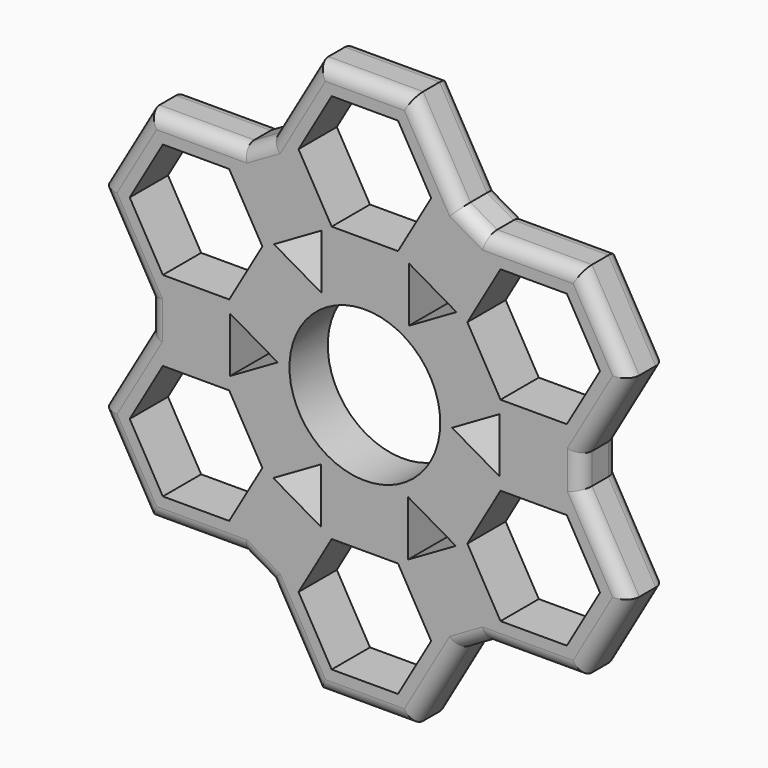
from build123d import *

# Parameters (mm, degrees)
F0_R     = 14.5
F0_R_2   = 11.025
F1_DEPTH = 7
F2_R     = 2
F4_DEPTH = 7


# Not quite as in the source:
# - a feature names something its author has since deleted; it is built from what else it names


with BuildPart() as f1:
    # F0 (on Front) → F1 (new body)
    with BuildSketch(Plane.XZ):
        Polygon((13.8564064606, 28.5096937621), (6.9282032303, 16.5096937621), (-6.9282032303, 16.5096937621), (-13.8564064606, 28.5096937621), (-17.7619158218, 26.254846881), (-10.8337125915, 14.254846881), (-17.7619158218, 2.254846881), (-31.6183222823, 2.254846881), (-31.6183222823, -2.254846881), (-17.7619158218, -2.254846881), (-10.8337125915, -14.254846881), (-17.7619158218, -26.254846881), (-13.8564064606, -28.5096937621), (-6.9282032303, -16.5096937621), (6.9282032303, -16.5096937621), (13.8564064606, -28.5096937621), (17.7619158218, -26.254846881), (10.8337125915, -14.254846881), (17.7619158218, -2.254846881), (31.6183222823, -2.254846881), (31.6183222823, 2.254846881), (17.7619158218, 2.254846881), (10.8337125915, 14.254846881), (17.7619158218, 26.254846881), align=None)
        Circle(F0_R, mode=Mode.SUBTRACT)
        Polygon((-6.9282032303, 16.5096937621), (6.9282032303, 16.5096937621), (13.8564064606, 28.5096937621), (6.9282032303, 40.5096937621), (-6.9282032303, 40.5096937621), (-13.8564064606, 28.5096937621), align=None)
        Polygon((9.6994845224, 28.5096937621), (4.8497422612, 20.1096937621), (-4.8497422612, 20.1096937621), (-9.6994845224, 28.5096937621), (-4.8497422612, 36.9096937621), (4.8497422612, 36.9096937621), align=None, mode=Mode.SUBTRACT)
        Polygon((31.6183222823, 26.254846881), (17.7619158218, 26.254846881), (10.8337125915, 14.254846881), (17.7619158218, 2.254846881), (31.6183222823, 2.254846881), (38.5465255126, 14.254846881), align=None)
        Polygon((29.5398613133, 22.654846881), (34.3896035744, 14.254846881), (29.5398613133, 5.854846881), (19.8403767909, 5.854846881), (14.9906345297, 14.254846881), (19.8403767909, 22.654846881), align=None, mode=Mode.SUBTRACT)
        Polygon((-10.8337125915, 14.254846881), (-17.7619158218, 26.254846881), (-31.6183222823, 26.254846881), (-38.5465255126, 14.254846881), (-31.6183222823, 2.254846881), (-17.7619158218, 2.254846881), align=None)
        Polygon((-34.3896035744, 14.254846881), (-29.5398613133, 22.654846881), (-19.8403767909, 22.654846881), (-14.9906345297, 14.254846881), (-19.8403767909, 5.854846881), (-29.5398613133, 5.854846881), align=None, mode=Mode.SUBTRACT)
        Polygon((38.5465255126, -14.254846881), (31.6183222823, -2.254846881), (17.7619158218, -2.254846881), (10.8337125915, -14.254846881), (17.7619158218, -26.254846881), (31.6183222823, -26.254846881), align=None)
        Polygon((34.3896035744, -14.254846881), (29.5398613133, -22.654846881), (19.8403767909, -22.654846881), (14.9906345297, -14.254846881), (19.8403767909, -5.854846881), (29.5398613133, -5.854846881), align=None, mode=Mode.SUBTRACT)
        Polygon((-17.7619158218, -2.254846881), (-31.6183222823, -2.254846881), (-38.5465255126, -14.254846881), (-31.6183222823, -26.254846881), (-17.7619158218, -26.254846881), (-10.8337125915, -14.254846881), align=None)
        Polygon((-29.5398613133, -22.654846881), (-34.3896035744, -14.254846881), (-29.5398613133, -5.854846881), (-19.8403767909, -5.854846881), (-14.9906345297, -14.254846881), (-19.8403767909, -22.654846881), align=None, mode=Mode.SUBTRACT)
        Polygon((6.9282032303, -40.5096937621), (13.8564064606, -28.5096937621), (6.9282032303, -16.5096937621), (-6.9282032303, -16.5096937621), (-13.8564064606, -28.5096937621), (-6.9282032303, -40.5096937621), align=None)
        Polygon((4.8497422612, -36.9096937621), (-4.8497422612, -36.9096937621), (-9.6994845224, -28.5096937621), (-4.8497422612, -20.1096937621), (4.8497422612, -20.1096937621), (9.6994845224, -28.5096937621), align=None, mode=Mode.SUBTRACT)
        Circle(F0_R)
        Circle(F0_R_2, mode=Mode.SUBTRACT)
    extrude(amount=F1_DEPTH)

    # F2
    f2_edges = [f1.edges().sort_by_distance(p)[0] for p in [
        (0, -7, 40.509694),
        (10.392305, -7, 34.509694),
        (24.690119, -7, 26.254847),
        (35.082424, -7, 20.254847),
        (35.082424, -7, 8.254847),
        (35.082424, -7, -8.254847),
        (35.082424, -7, -20.254847),
        (24.690119, -7, -26.254847),
        (10.392305, -7, -34.509694),
        (0, -7, -40.509694),
        (-10.392305, -7, -34.509694),
        (-24.690119, -7, -26.254847),
        (-35.082424, -7, -20.254847),
        (-35.082424, -7, -8.254847),
        (-35.082424, -7, 8.254847),
        (-35.082424, -7, 20.254847),
        (-24.690119, -7, 26.254847),
        (-10.392305, -7, 34.509694),
        (-10.392305, 0, -34.509694),
        (10.392305, 0, -34.509694),
        (24.690119, 0, -26.254847),
        (35.082424, 0, -20.254847),
        (35.082424, 0, -8.254847),
        (35.082424, 0, 8.254847),
        (35.082424, 0, 20.254847),
        (24.690119, 0, 26.254847),
        (10.392305, 0, 34.509694),
        (-24.690119, 0, 26.254847),
        (-35.082424, 0, 20.254847),
        (-35.082424, 0, 8.254847),
        (-35.082424, 0, -8.254847),
        (-35.082424, 0, -20.254847),
        (-24.690119, 0, -26.254847),
        (0, 0, -40.509694),
        (-10.392305, 0, 34.509694),
        (0, 0, 40.509694),
        (-15.809161, -7, 27.38227),
        (15.809161, -7, 27.38227),
        (31.618322, -7, 0),
        (15.809161, -7, -27.38227),
        (-15.809161, -7, -27.38227),
        (-31.618322, -7, 0),
        (-15.809161, 0, 27.38227),
        (15.809161, 0, 27.38227),
        (31.618322, 0, 0),
        (15.809161, 0, -27.38227),
        (-15.809161, 0, -27.38227),
        (-31.618322, 0, 0),
    ]]
    fillet(f2_edges, radius=F2_R)

    # F3 (on Front) → F4 (cut)
    with BuildSketch(Plane.XZ):
        Polygon((-6.3233720139, 11.0753334069), (-6.3233720139, 19.1219889618), (-13.2919801399, 15.0986611843), align=None)
        Polygon((-19.7218142187, 4.0847936793), (-19.7218142187, -3.9618618756), (-12.7532060927, 0.0614659018), align=None)
        Polygon((-13.3984422048, -15.0371952825), (-6.4298340788, -19.0605230599), (-6.4298340788, -11.013867505), align=None)
        Polygon((6.3233720139, -19.1219889618), (13.2919801399, -15.0986611843), (6.3233720139, -11.0753334069), align=None)
        Polygon((19.7218142187, -4.0847936793), (19.7218142187, 3.9618618756), (12.7532060927, -0.0614659018), align=None)
        Polygon((13.3984422048, 15.0371952825), (6.4298340788, 19.0605230599), (6.4298340788, 11.013867505), align=None)
    extrude(amount=F4_DEPTH, mode=Mode.SUBTRACT)


solid = f1.part
